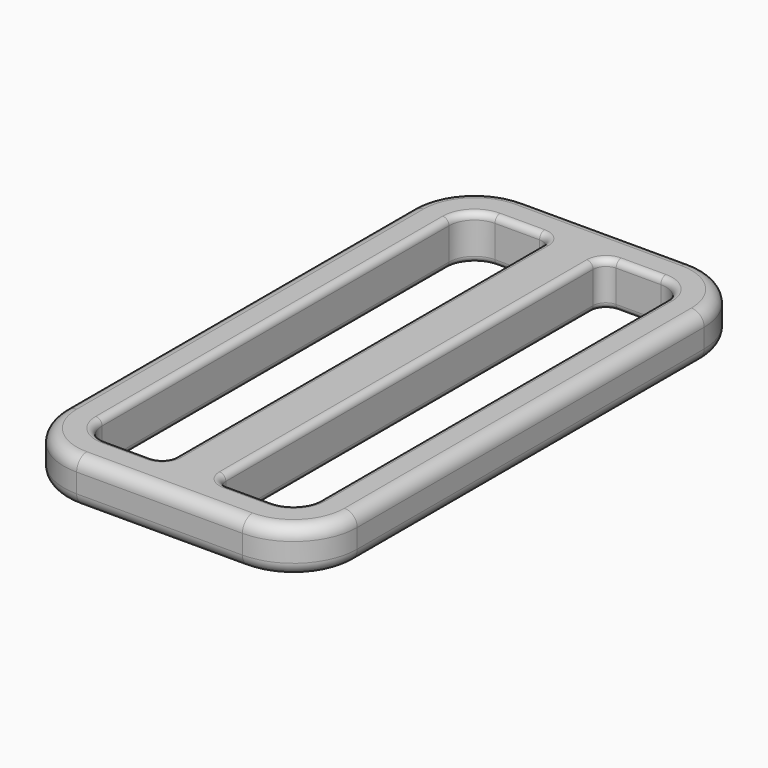
from build123d import *

# Parameters (mm, degrees)
F0_W     = 6.5
F0_H     = 38
F1_DEPTH = 3.5
F2_R     = 2
F3_R     = 1
F4_R     = 1
F5_R     = 0.5


with BuildPart() as f1:
    # F0 (on Top) → F1 (new body)
    with BuildSketch(Plane.XY):
        with BuildLine():
            Line((6.5, 22), (-6.5, 22))
            ThreePointArc((-6.5, 22), (-10.0355339059, 20.5355339059), (-11.5, 17))
            Line((-11.5, 17), (-11.5, -17))
            ThreePointArc((-11.5, -17), (-10.0355339059, -20.5355339059), (-6.5, -22))
            Line((-6.5, -22), (6.5, -22))
            ThreePointArc((6.5, -22), (10.0355339059, -20.5355339059), (11.5, -17))
            Line((11.5, -17), (11.5, 17))
            ThreePointArc((11.5, 17), (10.0355339059, 20.5355339059), (6.5, 22))
        make_face()
        with Locations((-5.25, 0)):
            Rectangle(F0_W, F0_H, mode=Mode.SUBTRACT)
        with Locations((5.25, 0)):
            Rectangle(F0_W, F0_H, mode=Mode.SUBTRACT)
    extrude(amount=F1_DEPTH)

    # F2
    f2_edges = [f1.edges().sort_by_distance(p)[0] for p in [
        (-8.5, 19, 1.75),
        (8.5, -19, 1.75),
        (8.5, 19, 1.75),
        (-8.5, -19, 1.75),
    ]]
    fillet(f2_edges, radius=F2_R)

    # F3
    f3_edges = [f1.edges().sort_by_distance(p)[0] for p in [
        (2, 19, 1.75),
        (-2, 19, 1.75),
        (-2, -19, 1.75),
        (2, -19, 1.75),
    ]]
    fillet(f3_edges, radius=F3_R)

    # F4
    f4_edges = [f1.edges().sort_by_distance(p)[0] for p in [
        (-11.5, 0, 3.5),
        (11.5, 0, 0),
        (10.035534, 20.535534, 0),
        (0, 22, 0),
        (-10.035534, 20.535534, 0),
        (-11.5, 0, 0),
        (-10.035534, -20.535534, 0),
        (0, -22, 0),
        (10.035534, -20.535534, 0),
        (10.035534, 20.535534, 3.5),
        (0, 22, 3.5),
        (-10.035534, 20.535534, 3.5),
        (-10.035534, -20.535534, 3.5),
        (0, -22, 3.5),
        (10.035534, -20.535534, 3.5),
        (11.5, 0, 3.5),
    ]]
    fillet(f4_edges, radius=F4_R)

    # F5
    f5_edges = [f1.edges().sort_by_distance(p)[0] for p in [
        (4.75, -19, 3.5),
        (-2.292893, -18.707107, 3.5),
        (-4.75, -19, 0),
        (4.75, -19, 0),
        (-2.292893, -18.707107, 0),
        (-7.914214, -18.414214, 0),
        (-2, 0, 0),
        (-8.5, 0, 0),
        (-2.292893, 18.707107, 0),
        (-7.914214, 18.414214, 0),
        (-4.75, 19, 0),
        (4.75, 19, 0),
        (2.292893, 18.707107, 0),
        (7.914214, 18.414214, 0),
        (2, 0, 0),
        (8.5, 0, 0),
        (2.292893, -18.707107, 0),
        (7.914214, -18.414214, 0),
        (-4.75, -19, 3.5),
        (-7.914214, -18.414214, 3.5),
        (-2, 0, 3.5),
        (-8.5, 0, 3.5),
        (-2.292893, 18.707107, 3.5),
        (-7.914214, 18.414214, 3.5),
        (-4.75, 19, 3.5),
        (4.75, 19, 3.5),
        (2.292893, 18.707107, 3.5),
        (7.914214, 18.414214, 3.5),
        (2, 0, 3.5),
        (8.5, 0, 3.5),
        (2.292893, -18.707107, 3.5),
        (7.914214, -18.414214, 3.5),
    ]]
    fillet(f5_edges, radius=F5_R)


solid = f1.part
